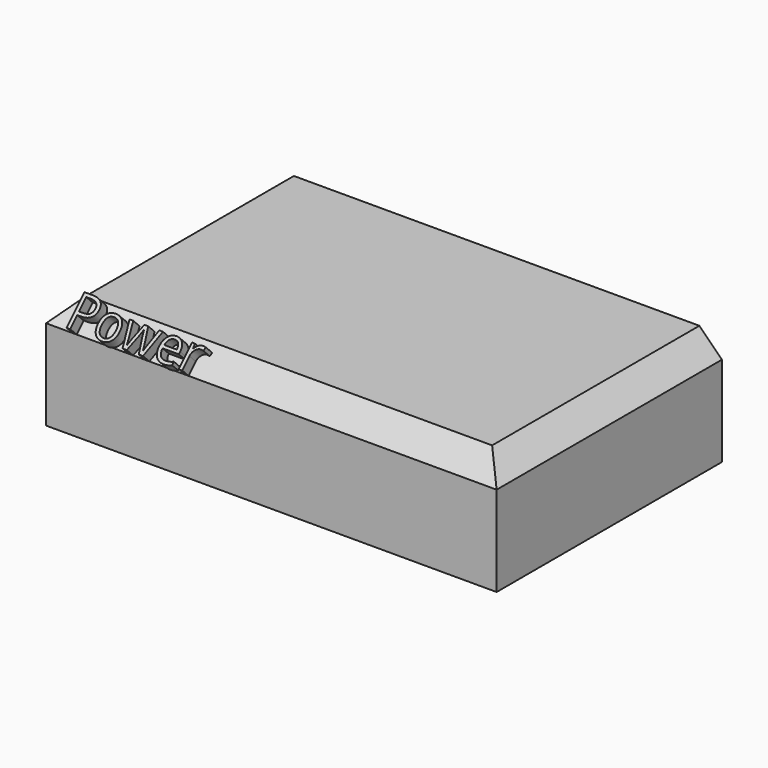
from build123d import *

# Parameters (mm, degrees)
F0_W         = 101.6
F0_H         = 63.5
F1_DEPTH     = 25.4
F2_SIZE      = 5.08
F3_TEXT_SIZE = 9.9780623567
F4_DEPTH     = 2.54


# Not quite as in the source:
# - Text() gives the source's letters only with a copy of the font that has no kerning and outlines rounded to 1/6400 em; it was checked with that copy


with BuildPart() as f1:
    # F0 (on Top) → F1 (new body)
    with BuildSketch(Plane.XY):
        Rectangle(F0_W, F0_H)
    extrude(amount=F1_DEPTH)

    # F2
    f2_edges = [f1.edges().sort_by_distance(p)[0] for p in [
        (50.8, 0, 25.4),
        (-50.8, 0, 25.4),
        (0, -31.75, 25.4),
    ]]
    chamfer(f2_edges, length=F2_SIZE)

    # F3 (on face) → F4 (join)
    with BuildSketch(Plane(origin=(0, -26.035, 26.035), x_dir=(1, 0, 0), z_dir=(0, -0.7071067812, 0.7071067812))):
        with Locations((-45.72, -8.082230509)):
            Text('Power', F3_TEXT_SIZE, font='Open Sans', text_align=(TextAlign.LEFT, TextAlign.BOTTOM))
    extrude(amount=F4_DEPTH)


solid = f1.part
